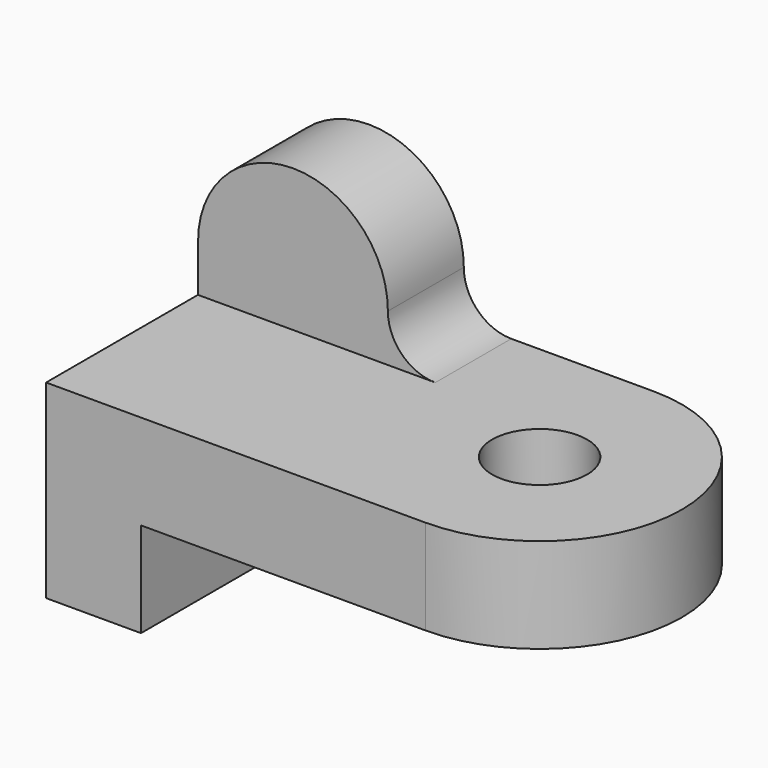
from build123d import *

# Parameters (mm, degrees)
F1_DEPTH = 12.7
F3_DEPTH = 12.7
F4_W     = 12.7
F4_H     = 38.1
F5_DEPTH = 12.7
F6_R     = 6.35
F7_DEPTH = 25.4
F8_R     = 6.34999


# Not quite as in the source:
# - a fillet or chamfer is up to 0.001 mm smaller than in the source, because OpenCascade refuses the exact size


with BuildPart() as f1:
    # F0 (on Top) → F1 (new body)
    with BuildSketch(Plane.XY):
        with BuildLine():
            ThreePointArc((29.6785237075, -38.1), (48.7285237075, -19.05), (29.6785237075, 0))
            Line((29.6785237075, 0), (-21.1214762925, 0))
            Line((-21.1214762925, 0), (-21.1214762925, -38.1))
            Line((-21.1214762925, -38.1), (29.6785237075, -38.1))
        make_face()
    extrude(amount=F1_DEPTH)

    # F2 (on Front) → F3 (join)
    with BuildSketch(Plane.XZ):
        with BuildLine():
            Line((-21.1026167169, 19.05), (-21.1026167169, 10.3077341521))
            Line((-21.1026167169, 10.3077341521), (4.2973832831, 10.3077341521))
            Line((4.2973832831, 10.3077341521), (4.2973832831, 19.05))
            ThreePointArc((4.2973832831, 19.05), (-8.4026167169, 31.75), (-21.1026167169, 19.05))
        make_face()
    extrude(amount=F3_DEPTH)

    # F4 (on face) → F5 (join)
    with BuildSketch(Plane.XY):
        with Locations((-14.7714762925, -19.05)):
            Rectangle(F4_W, F4_H)
    extrude(amount=-F5_DEPTH)

    # F6 (on face) → F7 (cut)
    with BuildSketch(Plane.XY.offset(12.7)):
        with Locations((29.6785237075, -19.05)):
            Circle(F6_R)
    extrude(amount=-F7_DEPTH, mode=Mode.SUBTRACT)

    # F8 (radius 6.35 in the source; OpenCascade refuses exactly that, so slightly less here)
    f8_edges = [f1.edges().sort_by_distance(p)[0] for p in [
        (4.297383, -6.35, 12.7),
    ]]
    fillet(f8_edges, radius=F8_R)


solid = f1.part
